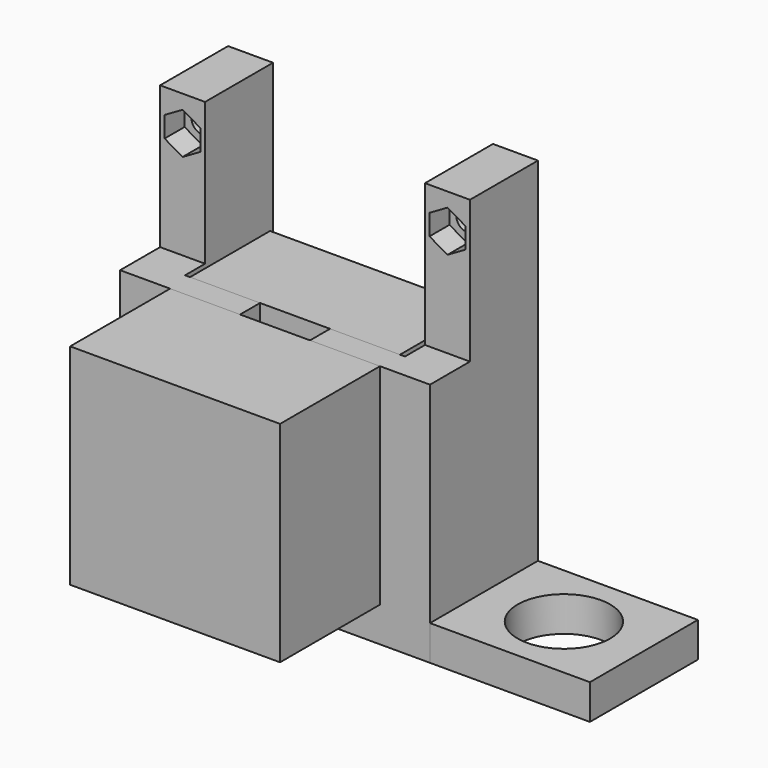
from build123d import *

# Parameters (mm, degrees)
F1_R      = 2.25
F2_DEPTH  = 12
F4_DEPTH  = 5
F5_W      = 44
F5_H      = 5
F6_DEPTH  = 7
F7_DEPTH  = 42
F8_R      = 1.7
F8_R_2    = 13
F9_DEPTH  = 5
F11_REACH = 63.8670687473
F12_R     = 1.7
F13_DEPTH = 20
F14_W     = 42
F14_H     = 42
F14_R     = 1.7
F14_R_2   = 13
F15_DEPTH = 25
F16_W     = 32
F16_H     = 27
F16_R     = 9.25
F17_DEPTH = 7


with BuildPart() as f2:
    # F1 (on Front) → F2 (new body)
    with BuildSketch(Plane.XZ):
        Polygon((-27, 56.5), (-36, 56.5), (-36, -21), (26, -21), (26, 56.5), (17, 56.5), (17, -14), (-27, -14), align=None)
        with Locations((-31.5, 49.5)):
            Circle(F1_R, mode=Mode.SUBTRACT)
        with Locations((21.5, 49.5)):
            Circle(F1_R, mode=Mode.SUBTRACT)
    extrude(amount=-F2_DEPTH)

    # F3 (on face) → F4 (join)
    with BuildSketch(Plane.XZ):
        Polygon((-27, -14), (-27, 56.5), (-36, 56.5), (-36, -21), (26, -21), (26, 56.5), (17, 56.5), (17, -14), align=None)
        Polygon((-31.5, 53.6569219382), (-27.9, 51.5784609691), (-27.9, 47.4215390309), (-31.5, 45.3430780618), (-35.1, 47.4215390309), (-35.1, 51.5784609691), align=None, mode=Mode.SUBTRACT)
        Polygon((21.5, 53.6569219382), (25.1, 51.5784609691), (25.1, 47.4215390309), (21.5, 45.3430780618), (17.9, 47.4215390309), (17.9, 51.5784609691), align=None, mode=Mode.SUBTRACT)
    extrude(amount=F4_DEPTH)

    # F5 (on face) → F6 (join, through all)
    with BuildSketch(Plane.XY.offset(-14)):
        with Locations((-5, -7.5)):
            Rectangle(F5_W, F5_H)
        with Locations((-5, -12.5)):
            Rectangle(F5_W, F5_H)
        Polygon((-27, -10), (-27, -5), (-36, -5), (-36, -15), (-27, -15), align=None)
        Polygon((26, -5), (17, -5), (17, -10), (17, -15), (26, -15), align=None)
    extrude(amount=-F6_DEPTH)

    # F5 (on face) → F7 (join)
    with BuildSketch(Plane.XY.offset(-14)):
        with Locations((-5, -12.5)):
            Rectangle(F5_W, F5_H)
        Polygon((-27, -10), (-27, -5), (-36, -5), (-36, -15), (-27, -15), align=None)
        Polygon((26, -5), (17, -5), (17, -10), (17, -15), (26, -15), align=None)
    extrude(amount=F7_DEPTH)

    # F8 (on face) → F9 (cut, through all)
    with BuildSketch(Plane.XZ.offset(15)):
        with Locations((-20.5, 22.5)):
            Circle(F8_R)
        with Locations((-5, 7)):
            Circle(F8_R_2)
        with Locations((-20.5, -8.5)):
            Circle(F8_R)
        with Locations((10.5, -8.5)):
            Circle(F8_R)
        with Locations((10.5, 22.5)):
            Circle(F8_R)
    extrude(amount=-F9_DEPTH, mode=Mode.SUBTRACT)

    f11_end = f2.faces().sort_by_distance((-18, -12.5, 7))[0]
    # F10 (on face) → F11 (cut, up to a face of the model that its end follows)
    with BuildSketch(Plane.XY.offset(28)):
        Polygon((2, -10), (-5, -10), (-12, -10), (-12, -15), (2, -15), align=None)
    f11_long = extrude(amount=-F11_REACH, mode=Mode.PRIVATE)
    add(split(f11_long, bisect_by=f11_end, keep=Keep.ALL, mode=Mode.PRIVATE).solids().sort_by_distance((-5, -12.5, 28))[0], mode=Mode.SUBTRACT)


with BuildPart() as f13:
    # F12 (on face) → F13 (new body)
    with BuildSketch(Plane(origin=(0, -10, 0), x_dir=(-1, 0, 0), z_dir=(0, 1, 0))):
        with BuildLine():
            Line((-16, -14), (26, -14))
            Line((26, -14), (26, 28))
            Line((26, 28), (12, 28))
            Line((12, 28), (12, 17.9544511501))
            ThreePointArc((12, 17.9544511501), (5, -6), (-2, 17.9544511501))
            Line((-2, 17.9544511501), (-2, 28))
            Line((-2, 28), (-16, 28))
            Line((-16, 28), (-16, -14))
        make_face()
        with Locations((-10.5, -8.5)):
            Circle(F12_R, mode=Mode.SUBTRACT)
        with Locations((20.5, -8.5)):
            Circle(F12_R, mode=Mode.SUBTRACT)
        with Locations((-10.5, 22.5)):
            Circle(F12_R, mode=Mode.SUBTRACT)
        with Locations((20.5, 22.5)):
            Circle(F12_R, mode=Mode.SUBTRACT)
        with BuildLine():
            Line((12, 17.9544511501), (12, 28))
            Line((12, 28), (-2, 28))
            Line((-2, 28), (-2, 17.9544511501))
            ThreePointArc((-2, 17.9544511501), (5, -6), (12, 17.9544511501))
        make_face()
        with Locations((-10.5, 22.5)):
            Circle(F12_R)
        with Locations((20.5, 22.5)):
            Circle(F12_R)
        with Locations((-10.5, -8.5)):
            Circle(F12_R)
        with Locations((20.5, -8.5)):
            Circle(F12_R)
    extrude(amount=F13_DEPTH)


with BuildPart() as f15:
    # F14 (on face) → F15 (new body)
    with BuildSketch(Plane.XZ.offset(15)):
        with Locations((-5, 7)):
            Rectangle(F14_W, F14_H)
        with Locations((-20.5, -8.5)):
            Circle(F14_R, mode=Mode.SUBTRACT)
        with Locations((10.5, -8.5)):
            Circle(F14_R, mode=Mode.SUBTRACT)
        with Locations((-20.5, 22.5)):
            Circle(F14_R, mode=Mode.SUBTRACT)
        with Locations((-5, 7)):
            Circle(F14_R_2, mode=Mode.SUBTRACT)
        with Locations((10.5, 22.5)):
            Circle(F14_R, mode=Mode.SUBTRACT)
    extrude(amount=F15_DEPTH)

    # F8 (on face) → F15, piece 2 (join)
    with BuildSketch(Plane.XZ.offset(15)):
        with Locations((-20.5, 22.5)):
            Circle(F8_R)
    extrude(amount=F15_DEPTH)

    # F8 (on face) → F15, piece 3 (join)
    with BuildSketch(Plane.XZ.offset(15)):
        with Locations((-5, 7)):
            Circle(F8_R_2)
    extrude(amount=F15_DEPTH)

    # F8 (on face) → F15, piece 4 (join)
    with BuildSketch(Plane.XZ.offset(15)):
        with Locations((-20.5, -8.5)):
            Circle(F8_R)
    extrude(amount=F15_DEPTH)

    # F8 (on face) → F15, piece 5 (join)
    with BuildSketch(Plane.XZ.offset(15)):
        with Locations((10.5, 22.5)):
            Circle(F8_R)
    extrude(amount=F15_DEPTH)

    # F8 (on face) → F15, piece 6 (join)
    with BuildSketch(Plane.XZ.offset(15)):
        with Locations((10.5, -8.5)):
            Circle(F8_R)
    extrude(amount=F15_DEPTH)


with BuildPart() as f17:
    # F16 (on face) → F17 (new body, through all)
    with BuildSketch(Plane(origin=(0, 0, -21), x_dir=(1, 0, 0), z_dir=(0, 0, -1))):
        with Locations((42, 1.5)):
            Rectangle(F16_W, F16_H)
        with Locations((42, 1.5)):
            Circle(F16_R, mode=Mode.SUBTRACT)
    extrude(amount=-F17_DEPTH)


solid = Compound([f2.part, f13.part, f15.part, f17.part])
